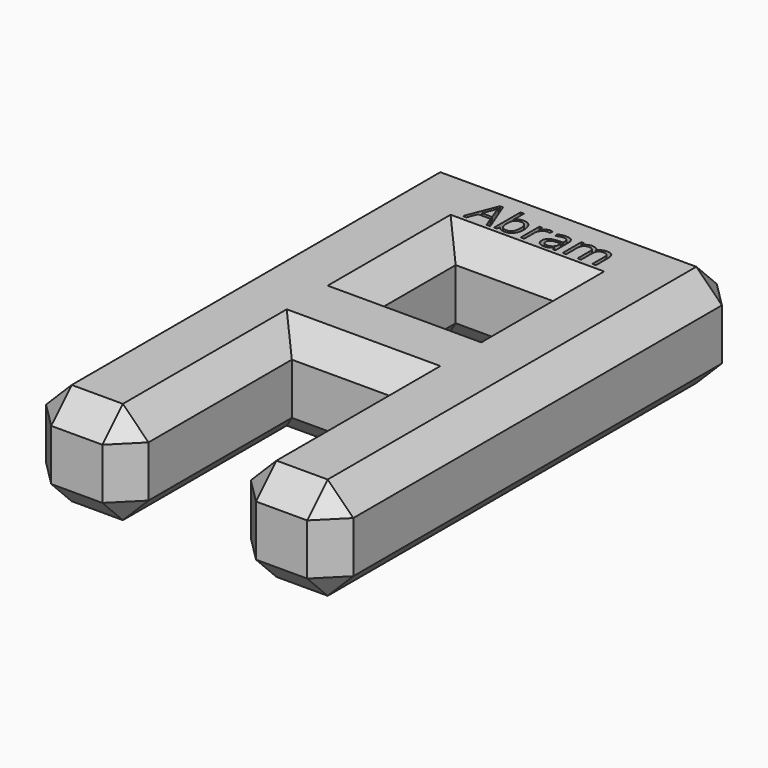
from build123d import *

# Parameters (mm, degrees)
F0_W         = 15.24
F0_H         = 25.4
F1_DEPTH     = 5.08
F2_W         = 5.08
F2_H         = 5.08
F2_H_2       = 10.16
F3_DEPTH     = 5.08
F5_SIZE      = 1.27
F4_TEXT_SIZE = 2.158443547
F6_DEPTH     = 1.27


# Not quite as in the source:
# - Text() gives the source's letters only with a copy of the font that has no kerning and outlines rounded to 1/6400 em; it was checked with that copy


with BuildPart() as f1:
    # F0 (on Top) → F1 (new body)
    with BuildSketch(Plane.XY):
        Rectangle(F0_W, F0_H)
    extrude(amount=F1_DEPTH)

    # F2 (on face) → F3 (cut)
    with BuildSketch(Plane.XY.offset(5.08)):
        with Locations((0, 5.08)):
            Rectangle(F2_W, F2_H)
        with Locations((0, -7.62)):
            Rectangle(F2_W, F2_H_2)
    extrude(amount=-F3_DEPTH, mode=Mode.SUBTRACT)

    # F5
    f5_edges = [f1.edges().sort_by_distance(p)[0] for p in [
        (0, 2.54, 5.08),
        (-2.54, 5.08, 5.08),
        (2.54, 5.08, 5.08),
        (0, 7.62, 5.08),
        (0, 2.54, 0),
        (2.54, 5.08, 0),
        (0, 7.62, 0),
        (-2.54, 5.08, 0),
        (0, 12.7, 0),
        (0, 12.7, 5.08),
        (0, -2.54, 0),
        (0, -2.54, 5.08),
        (-5.08, -12.7, 5.08),
        (5.08, -12.7, 0),
        (-5.08, -12.7, 0),
        (5.08, -12.7, 5.08),
        (7.62, 0, 0),
        (-7.62, 0, 0),
        (7.62, 0, 5.08),
        (-7.62, 0, 5.08),
        (-2.54, -7.62, 5.08),
        (2.54, -7.62, 5.08),
        (-2.54, -7.62, 0),
        (2.54, -7.62, 0),
        (-7.62, 12.7, 2.54),
        (7.62, 12.7, 2.54),
        (7.62, -12.7, 2.54),
        (2.54, -12.7, 2.54),
        (-2.54, -12.7, 2.54),
        (-7.62, -12.7, 2.54),
    ]]
    chamfer(f5_edges, length=F5_SIZE)

    # F4 (on face) → F6 (cut)
    with BuildSketch(Plane.XY.offset(5.08)):
        with Locations((-3.3713876433, 9.0988809243)):
            Text('Abram', F4_TEXT_SIZE, font='Open Sans', text_align=(TextAlign.LEFT, TextAlign.BOTTOM))
    extrude(amount=-F6_DEPTH, mode=Mode.SUBTRACT)


solid = f1.part
